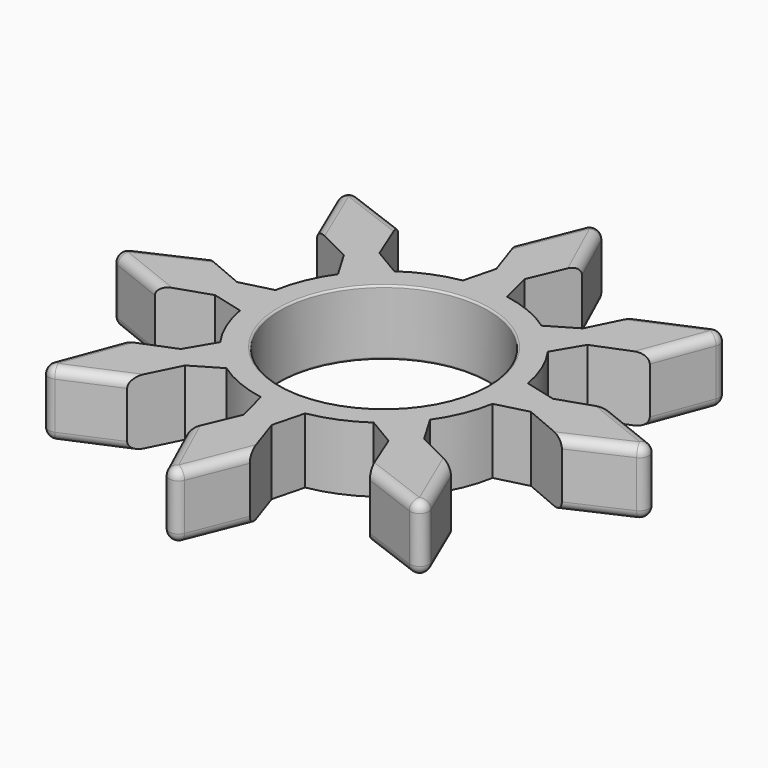
from build123d import *

# Parameters (mm, degrees)
F0_R         = 11.15
F1_DEPTH     = 7
F2_T1_DEPTH  = 13.6241967353
F2_T3_DEPTH  = 13.6241967353
F2_T5_DEPTH  = 13.6241967353
F2_T7_DEPTH  = 13.6241967353
F2_T9_DEPTH  = 13.6241967353
F2_T11_DEPTH = 13.6241967353
F2_T13_DEPTH = 13.6241967353
F3_T1_DEPTH  = 8.9632694004
F3_T3_DEPTH  = 8.9632694004
F3_T5_DEPTH  = 8.9632694004
F3_T7_DEPTH  = 8.9632694004
F3_T9_DEPTH  = 8.9632694004
F3_T11_DEPTH = 8.9632694004
F3_T13_DEPTH = 13.8051316922
F3_T15_DEPTH = 8.9632694004
F3_T17_DEPTH = 11.8546557295
F3_T22_DEPTH = 1
F3_T28_DEPTH = 1
F3_T34_DEPTH = 1
F3_T40_DEPTH = 1
F3_T46_DEPTH = 1
F3_T52_DEPTH = 1
F3_T58_DEPTH = 1
F4_R         = 1
F5_T1_DEPTH  = 8.7823344436
F5_T3_DEPTH  = 5
F5_T8_DEPTH  = 1
F5_T14_DEPTH = 1
F6_R         = 0.2


# Not quite as in the source:
# - a fillet or chamfer that OpenCascade refuses, or shapes differently, is made with other operations: its cross-section is extruded or revolved along the edge and cut away or added


with BuildPart() as f1:
    # F0 (on Top) → F1 (new body)
    with BuildSketch(Plane.XY):
        with BuildLine():
            ThreePointArc((2.3756959996, 13.5358058293), (0.0020367359, 13.7427059484), (-2.3716837507, 13.5365094141))
            ThreePointArc((-2.3716837507, 13.5365094141), (-5.2572241837, 12.6973841721), (-7.8913893394, 11.2511308421))
            ThreePointArc((-7.8913893394, 11.2511308421), (-9.7161203782, 9.7190007577), (-11.2487912633, 7.8947239373))
            ThreePointArc((-11.2487912633, 7.8947239373), (-12.695825322, 5.2609875809), (-13.5358058293, 2.3756959996))
            ThreePointArc((-13.5358058293, 2.3756959996), (-13.7427059484, 0.0020367359), (-13.5365094141, -2.3716837507))
            ThreePointArc((-13.5365094141, -2.3716837507), (-12.6973841721, -5.2572241837), (-11.2511308421, -7.8913893394))
            ThreePointArc((-11.2511308421, -7.8913893394), (-9.7190007577, -9.7161203782), (-7.8947239373, -11.2487912633))
            ThreePointArc((-7.8947239373, -11.2487912633), (-5.2609875809, -12.695825322), (-2.3756959996, -13.5358058293))
            ThreePointArc((-2.3756959996, -13.5358058293), (-0.0020367359, -13.7427059484), (2.3716837507, -13.5365094141))
            ThreePointArc((2.3716837507, -13.5365094141), (5.2572241837, -12.6973841721), (7.8913893394, -11.2511308421))
            ThreePointArc((7.8913893394, -11.2511308421), (9.7161203782, -9.7190007577), (11.2487912633, -7.8947239373))
            ThreePointArc((11.2487912633, -7.8947239373), (12.695825322, -5.2609875809), (13.5358058293, -2.3756959996))
            ThreePointArc((13.5358058293, -2.3756959996), (13.6908833218, -1.192344246), (13.7427060993, 0))
            ThreePointArc((13.7427060993, 0), (13.6910598827, 1.1903151774), (13.5365094141, 2.3716837507))
            ThreePointArc((13.5365094141, 2.3716837507), (12.6973841721, 5.2572241837), (11.2511308421, 7.8913893394))
            ThreePointArc((11.2511308421, 7.8913893394), (9.7190007577, 9.7161203782), (7.8947239373, 11.2487912633))
            ThreePointArc((7.8947239373, 11.2487912633), (5.2609875809, 12.695825322), (2.3756959996, 13.5358058293))
        make_face()
        Circle(F0_R, mode=Mode.SUBTRACT)
        with BuildLine():
            ThreePointArc((-13.5365094141, -2.3716837507), (-13.7427059484, 0.0020367359), (-13.5358058293, 2.3756959996))
            Line((-13.5358058293, 2.3756959996), (-16.9547849556, 1.5))
            Line((-16.9547849556, 1.5), (-21.9830603232, 3.6412940468))
            Line((-21.9830603232, 3.6412940468), (-30, 0))
            Line((-30, 0), (-21.9935868419, -3.2053264533))
            Line((-21.9935868419, -3.2053264533), (-16.923192294, -1.4996672643))
            Line((-16.923192294, -1.4996672643), (-13.5365094141, -2.3716837507))
        make_face()
        with BuildLine():
            ThreePointArc((-11.2487912633, 7.8947239373), (-9.7161203782, 9.7190007577), (-7.8913893394, 11.2511308421))
            Line((-7.8913893394, 11.2511308421), (-10.9281832439, 13.0495035874))
            Line((-10.9281832439, 13.0495035874), (-12.969587313, 18.1191547385))
            Line((-12.969587313, 18.1191547385), (-21.2132034356, 21.2132034356))
            Line((-21.2132034356, 21.2132034356), (-17.8183224696, 13.2853063275))
            Line((-17.8183224696, 13.2853063275), (-13.0269289226, 10.9060791383))
            Line((-13.0269289226, 10.9060791383), (-11.2487912633, 7.8947239373))
        make_face()
        with BuildLine():
            Line((3.6412940468, 21.9830603232), (0, 30))
            Line((0, 30), (-3.2053264533, 21.9935868419))
            Line((-3.2053264533, 21.9935868419), (-1.4996672643, 16.923192294))
            Line((-1.4996672643, 16.923192294), (-2.3716837507, 13.5365094141))
            ThreePointArc((-2.3716837507, 13.5365094141), (0.0020367359, 13.7427059484), (2.3756959996, 13.5358058293))
            Line((2.3756959996, 13.5358058293), (1.5, 16.9547849556))
            Line((1.5, 16.9547849556), (3.6412940468, 21.9830603232))
        make_face()
        with BuildLine():
            Line((10.9060791383, 13.0269289226), (7.8947239373, 11.2487912633))
            ThreePointArc((7.8947239373, 11.2487912633), (9.7190007577, 9.7161203782), (11.2511308421, 7.8913893394))
            Line((11.2511308421, 7.8913893394), (13.0495035874, 10.9281832439))
            Line((13.0495035874, 10.9281832439), (18.1191547385, 12.969587313))
            Line((18.1191547385, 12.969587313), (21.2132034356, 21.2132034356))
            Line((21.2132034356, 21.2132034356), (13.2853063275, 17.8183224696))
            Line((13.2853063275, 17.8183224696), (10.9060791383, 13.0269289226))
        make_face()
        with BuildLine():
            Line((16.923192294, 1.4996672643), (13.5365094141, 2.3716837507))
            ThreePointArc((13.5365094141, 2.3716837507), (13.6910598827, 1.1903151774), (13.7427060993, 0))
            ThreePointArc((13.7427060993, 0), (13.6908833218, -1.192344246), (13.5358058293, -2.3756959996))
            Line((13.5358058293, -2.3756959996), (16.9547849556, -1.5))
            Line((16.9547849556, -1.5), (21.9830603232, -3.6412940468))
            Line((21.9830603232, -3.6412940468), (30, 0))
            Line((30, 0), (21.9935868419, 3.2053264533))
            Line((21.9935868419, 3.2053264533), (16.923192294, 1.4996672643))
        make_face()
        with BuildLine():
            Line((13.0269289226, -10.9060791383), (11.2487912633, -7.8947239373))
            ThreePointArc((11.2487912633, -7.8947239373), (9.7161203782, -9.7190007577), (7.8913893394, -11.2511308421))
            Line((7.8913893394, -11.2511308421), (10.9281832439, -13.0495035874))
            Line((10.9281832439, -13.0495035874), (12.969587313, -18.1191547385))
            Line((12.969587313, -18.1191547385), (21.2132034356, -21.2132034356))
            Line((21.2132034356, -21.2132034356), (17.8183224696, -13.2853063275))
            Line((17.8183224696, -13.2853063275), (13.0269289226, -10.9060791383))
        make_face()
        with BuildLine():
            ThreePointArc((2.3716837507, -13.5365094141), (-0.0020367359, -13.7427059484), (-2.3756959996, -13.5358058293))
            Line((-2.3756959996, -13.5358058293), (-1.5, -16.9547849556))
            Line((-1.5, -16.9547849556), (-3.6412940468, -21.9830603232))
            Line((-3.6412940468, -21.9830603232), (0, -30))
            Line((0, -30), (3.2053264533, -21.9935868419))
            Line((3.2053264533, -21.9935868419), (1.4996672643, -16.923192294))
            Line((1.4996672643, -16.923192294), (2.3716837507, -13.5365094141))
        make_face()
        with BuildLine():
            ThreePointArc((-7.8947239373, -11.2487912633), (-9.7190007577, -9.7161203782), (-11.2511308421, -7.8913893394))
            Line((-11.2511308421, -7.8913893394), (-13.0495035874, -10.9281832439))
            Line((-13.0495035874, -10.9281832439), (-18.1191547385, -12.969587313))
            Line((-18.1191547385, -12.969587313), (-21.2132034356, -21.2132034356))
            Line((-21.2132034356, -21.2132034356), (-13.2853063275, -17.8183224696))
            Line((-13.2853063275, -17.8183224696), (-10.9060791383, -13.0269289226))
            Line((-10.9060791383, -13.0269289226), (-7.8947239373, -11.2487912633))
        make_face()
    extrude(amount=F1_DEPTH)

    # F2: fillet of radius 1 on 7 edges, made by hand

    # F2_s2 → F2_t1 (cut)
    with BuildSketch(Plane(origin=(-28.1768322846, 11.2804503226, 0), x_dir=(0, 0, 1), z_dir=(0.9283662472, -0.3716666667, 0))):
        with BuildLine():
            ThreePointArc((6, 11.15), (6.7071067812, 10.8571067812), (7, 10.15))
            Line((7, 10.15), (7, 11.15))
            Line((7, 11.15), (6, 11.15))
        make_face()
    extrude(amount=F2_T1_DEPTH, mode=Mode.SUBTRACT)

    # F2_s4 → F2_t3 (cut)
    with BuildSketch(Plane(origin=(-11.9475462628, 27.9005120988, 0), x_dir=(0, 0, 1), z_dir=(0.3936460485, -0.9192620891, 0))):
        with BuildLine():
            ThreePointArc((6, 11.15), (6.7071067812, 10.8571067812), (7, 10.15))
            Line((7, 10.15), (7, 11.15))
            Line((7, 11.15), (6, 11.15))
        make_face()
    extrude(amount=F2_T3_DEPTH, mode=Mode.SUBTRACT)

    # F2_s6 → F2_t5 (cut)
    with BuildSketch(Plane(origin=(11.2804503226, 28.1768322846, 0), x_dir=(0, 0, 1), z_dir=(-0.3716666667, -0.9283662472, 0))):
        with BuildLine():
            ThreePointArc((6, 11.15), (6.7071067812, 10.8571067812), (7, 10.15))
            Line((7, 10.15), (7, 11.15))
            Line((7, 11.15), (6, 11.15))
        make_face()
    extrude(amount=F2_T5_DEPTH, mode=Mode.SUBTRACT)

    # F2_s8 → F2_t7 (cut)
    with BuildSketch(Plane(origin=(27.9005120988, 11.9475462628, 0), x_dir=(0, 0, 1), z_dir=(-0.9192620891, -0.3936460485, 0))):
        with BuildLine():
            ThreePointArc((6, 11.15), (6.7071067812, 10.8571067812), (7, 10.15))
            Line((7, 10.15), (7, 11.15))
            Line((7, 11.15), (6, 11.15))
        make_face()
    extrude(amount=F2_T7_DEPTH, mode=Mode.SUBTRACT)

    # F2_s10 → F2_t9 (cut)
    with BuildSketch(Plane(origin=(28.1768322846, -11.2804503226, 0), x_dir=(0, 0, 1), z_dir=(-0.9283662472, 0.3716666667, 0))):
        with BuildLine():
            ThreePointArc((6, 11.15), (6.7071067812, 10.8571067812), (7, 10.15))
            Line((7, 10.15), (7, 11.15))
            Line((7, 11.15), (6, 11.15))
        make_face()
    extrude(amount=F2_T9_DEPTH, mode=Mode.SUBTRACT)

    # F2_s12 → F2_t11 (cut)
    with BuildSketch(Plane(origin=(11.9475462628, -27.9005120988, 0), x_dir=(0, 0, 1), z_dir=(-0.3936460485, 0.9192620891, 0))):
        with BuildLine():
            ThreePointArc((6, 11.15), (6.7071067812, 10.8571067812), (7, 10.15))
            Line((7, 10.15), (7, 11.15))
            Line((7, 11.15), (6, 11.15))
        make_face()
    extrude(amount=F2_T11_DEPTH, mode=Mode.SUBTRACT)

    # F2_s14 → F2_t13 (cut)
    with BuildSketch(Plane(origin=(-11.2804503226, -28.1768322846, 0), x_dir=(0, 0, 1), z_dir=(0.3716666667, 0.9283662472, 0))):
        with BuildLine():
            ThreePointArc((6, 11.15), (6.7071067812, 10.8571067812), (7, 10.15))
            Line((7, 10.15), (7, 11.15))
            Line((7, 11.15), (6, 11.15))
        make_face()
    extrude(amount=F2_T13_DEPTH, mode=Mode.SUBTRACT)

    # F3: fillet of radius 1 on 8 edges, made by hand

    # F3_s2 → F3_t1 (cut)
    with BuildSketch(Plane(origin=(-14.9884732198, 5.6255732129, 0), x_dir=(0, 0, 1), z_dir=(-0.9362286006, 0.35139153, 0))):
        with BuildLine():
            ThreePointArc((7, 11.4062677563), (6.7071067812, 12.1133745375), (6, 12.4062677563))
            Line((6, 12.4062677563), (7, 12.4062677563))
            Line((7, 12.4062677563), (7, 11.4062677563))
        make_face()
    extrude(amount=F3_T1_DEPTH, mode=Mode.SUBTRACT)

    # F3_s4 → F3_t3 (cut)
    with BuildSketch(Plane(origin=(-6.6205700864, 14.5763320202, 0), x_dir=(0, 0, 1), z_dir=(-0.4135422585, 0.910484926, 0))):
        with BuildLine():
            ThreePointArc((7, 11.4062677563), (6.7071067812, 12.1133745375), (6, 12.4062677563))
            Line((6, 12.4062677563), (7, 12.4062677563))
            Line((7, 12.4062677563), (7, 11.4062677563))
        make_face()
    extrude(amount=F3_T3_DEPTH, mode=Mode.SUBTRACT)

    # F3_s6 → F3_t5 (cut)
    with BuildSketch(Plane(origin=(5.6255732129, 14.9884732198, 0), x_dir=(0, 0, 1), z_dir=(0.35139153, 0.9362286006, 0))):
        with BuildLine():
            ThreePointArc((7, 11.4062677563), (6.7071067812, 12.1133745375), (6, 12.4062677563))
            Line((6, 12.4062677563), (7, 12.4062677563))
            Line((7, 12.4062677563), (7, 11.4062677563))
        make_face()
    extrude(amount=F3_T5_DEPTH, mode=Mode.SUBTRACT)

    # F3_s8 → F3_t7 (cut)
    with BuildSketch(Plane(origin=(14.5763320202, 6.6205700864, 0), x_dir=(0, 0, 1), z_dir=(0.910484926, 0.4135422585, 0))):
        with BuildLine():
            ThreePointArc((7, 11.4062677563), (6.7071067812, 12.1133745375), (6, 12.4062677563))
            Line((6, 12.4062677563), (7, 12.4062677563))
            Line((7, 12.4062677563), (7, 11.4062677563))
        make_face()
    extrude(amount=F3_T7_DEPTH, mode=Mode.SUBTRACT)

    # F3_s10 → F3_t9 (cut)
    with BuildSketch(Plane(origin=(14.9884732198, -5.6255732129, 0), x_dir=(0, 0, 1), z_dir=(0.9362286006, -0.35139153, 0))):
        with BuildLine():
            ThreePointArc((7, 11.4062677563), (6.7071067812, 12.1133745375), (6, 12.4062677563))
            Line((6, 12.4062677563), (7, 12.4062677563))
            Line((7, 12.4062677563), (7, 11.4062677563))
        make_face()
    extrude(amount=F3_T9_DEPTH, mode=Mode.SUBTRACT)

    # F3_s12 → F3_t11 (cut)
    with BuildSketch(Plane(origin=(6.6205700864, -14.5763320202, 0), x_dir=(0, 0, 1), z_dir=(0.4135422585, -0.910484926, 0))):
        with BuildLine():
            ThreePointArc((7, 11.4062677563), (6.7071067812, 12.1133745375), (6, 12.4062677563))
            Line((6, 12.4062677563), (7, 12.4062677563))
            Line((7, 12.4062677563), (7, 11.4062677563))
        make_face()
    extrude(amount=F3_T11_DEPTH, mode=Mode.SUBTRACT)

    # F3_s14 → F3_t13 (cut)
    with BuildSketch(Plane(origin=(-5.6255732129, -14.9884732198, 0), x_dir=(0, 0, 1), z_dir=(-0.35139153, -0.9362286006, 0))):
        with BuildLine():
            ThreePointArc((7, 11.4062677563), (6.7071067812, 12.1133745375), (6, 12.4062677563))
            Line((6, 12.4062677563), (7, 12.4062677563))
            Line((7, 12.4062677563), (7, 11.4062677563))
        make_face()
    extrude(amount=F3_T13_DEPTH, mode=Mode.SUBTRACT)

    # F3_s16 → F3_t15 (cut)
    with BuildSketch(Plane(origin=(-14.5763320202, -6.6205700864, 0), x_dir=(0, 0, 1), z_dir=(-0.910484926, -0.4135422585, 0))):
        with BuildLine():
            ThreePointArc((7, 11.4062677563), (6.7071067812, 12.1133745375), (6, 12.4062677563))
            Line((6, 12.4062677563), (7, 12.4062677563))
            Line((7, 12.4062677563), (7, 11.4062677563))
        make_face()
    extrude(amount=F3_T15_DEPTH, mode=Mode.SUBTRACT)

    # F3_s18 → F3_t17 (cut)
    with BuildSketch(Plane.XY.offset(-5.8546557295)):
        with BuildLine():
            ThreePointArc((-27.8677696847, 0.9684590213), (-28.4539682292, 0.0352073057), (-27.8258940928, -0.8703921518))
            Line((-27.8258940928, -0.8703921518), (-30, 0))
            Line((-30, 0), (-27.8677696847, 0.9684590213))
        make_face()
        with BuildLine():
            ThreePointArc((-0.9684590213, -27.8677696847), (-0.0352073057, -28.4539682292), (0.8703921518, -27.8258940928))
            Line((0.8703921518, -27.8258940928), (0, -30))
            Line((0, -30), (-0.9684590213, -27.8677696847))
        make_face()
        with BuildLine():
            ThreePointArc((19.0206849793, -20.3902928619), (20.0950985619, -20.1448892111), (20.2913385984, -19.0604182128))
            Line((20.2913385984, -19.0604182128), (21.2132034356, -21.2132034356))
            Line((21.2132034356, -21.2132034356), (19.0206849793, -20.3902928619))
        make_face()
        with BuildLine():
            ThreePointArc((27.8677696847, -0.9684590213), (28.4539682292, -0.0352073057), (27.8258940928, 0.8703921518))
            Line((27.8258940928, 0.8703921518), (30, 0))
            Line((30, 0), (27.8677696847, -0.9684590213))
        make_face()
        with BuildLine():
            ThreePointArc((20.3902928619, 19.0206849793), (20.1448892111, 20.0950985619), (19.0604182128, 20.2913385984))
            Line((19.0604182128, 20.2913385984), (21.2132034356, 21.2132034356))
            Line((21.2132034356, 21.2132034356), (20.3902928619, 19.0206849793))
        make_face()
        with BuildLine():
            ThreePointArc((0.9684590213, 27.8677696847), (0.0352073057, 28.4539682292), (-0.8703921518, 27.8258940928))
            Line((-0.8703921518, 27.8258940928), (0, 30))
            Line((0, 30), (0.9684590213, 27.8677696847))
        make_face()
        with BuildLine():
            ThreePointArc((-19.0206849793, 20.3902928619), (-20.0950985619, 20.1448892111), (-20.2913385984, 19.0604182128))
            Line((-20.2913385984, 19.0604182128), (-21.2132034356, 21.2132034356))
            Line((-21.2132034356, 21.2132034356), (-19.0206849793, 20.3902928619))
        make_face()
    extrude(amount=F3_T17_DEPTH, mode=Mode.SUBTRACT)


with BuildPart() as f3_tool20:
    # F3_s21 → F3_t22 (new body)
    with BuildSketch(Plane.XY.offset(6)):
        Polygon((-27.4542274261, 0.0579740954), (-27.8677696847, 0.9684590213), (-30, 0), (-27.8258940928, -0.8703921518), align=None)
    extrude(amount=F3_T22_DEPTH)

    # F3_s23 → F3_t24 (revolve, cut)
    with BuildSketch(Plane(origin=(-27.4542274261, 0.0579740954, 6), x_dir=(0.9997408031, 0.0227667896, 0), z_dir=(0.0227667896, -0.9997408031, 0))):
        with BuildLine():
            ThreePointArc((0, -1), (1, 0), (0, 1))
            Line((0, 1), (0, -1))
        make_face()
    revolve(axis=Axis((-27.4542274261, 0.0579740954, 6), (0, 0, 1)), mode=Mode.SUBTRACT)


with BuildPart() as f1_1:
    add(f1.part)

    # F3_t19: cut F3_tool20
    add(f3_tool20.part, mode=Mode.SUBTRACT)


with BuildPart() as f3_tool26:
    # F3_s27 → F3_t28 (new body)
    with BuildSketch(Plane.XY.offset(6)):
        Polygon((-0.0579740954, -27.4542274261), (-0.9684590213, -27.8677696847), (0, -30), (0.8703921518, -27.8258940928), align=None)
    extrude(amount=F3_T28_DEPTH)

    # F3_s29 → F3_t30 (revolve, cut)
    with BuildSketch(Plane(origin=(-0.0579740954, -27.4542274261, 6), x_dir=(-0.0227667896, 0.9997408031, 0), z_dir=(0.9997408031, 0.0227667896, 0))):
        with BuildLine():
            ThreePointArc((0, -1), (1, 0), (0, 1))
            Line((0, 1), (0, -1))
        make_face()
    revolve(axis=Axis((-0.0579740954, -27.4542274261, 6), (0, 0, 1)), mode=Mode.SUBTRACT)


with BuildPart() as f1_2:
    add(f1_1.part)

    # F3_t25: cut F3_tool26
    add(f3_tool26.part, mode=Mode.SUBTRACT)


with BuildPart() as f3_tool32:
    # F3_s33 → F3_t34 (new body)
    with BuildSketch(Plane.XY.offset(6)):
        Polygon((19.3720765093, -19.4540642612), (20.2913385984, -19.0604182128), (21.2132034356, -21.2132034356), (19.0206849793, -20.3902928619), align=None)
    extrude(amount=F3_T34_DEPTH)

    # F3_s35 → F3_t36 (revolve, cut)
    with BuildSketch(Plane(origin=(19.3720765093, -19.4540642612, 6), x_dir=(-0.7230220526, 0.6908249499, 0), z_dir=(0.6908249499, 0.7230220526, 0))):
        with BuildLine():
            ThreePointArc((0, -1), (1, 0), (0, 1))
            Line((0, 1), (0, -1))
        make_face()
    revolve(axis=Axis((19.3720765093, -19.4540642612, 6), (0, 0, 1)), mode=Mode.SUBTRACT)


with BuildPart() as f1_3:
    add(f1_2.part)

    # F3_t31: cut F3_tool32
    add(f3_tool32.part, mode=Mode.SUBTRACT)


with BuildPart() as f3_tool38:
    # F3_s39 → F3_t40 (new body)
    with BuildSketch(Plane.XY.offset(6)):
        Polygon((27.4542274261, -0.0579740954), (27.8677696847, -0.9684590213), (30, 0), (27.8258940928, 0.8703921518), align=None)
    extrude(amount=F3_T40_DEPTH)

    # F3_s41 → F3_t42 (revolve, cut)
    with BuildSketch(Plane(origin=(27.4542274261, -0.0579740954, 6), x_dir=(-0.9997408031, -0.0227667896, 0), z_dir=(-0.0227667896, 0.9997408031, 0))):
        with BuildLine():
            ThreePointArc((0, -1), (1, 0), (0, 1))
            Line((0, 1), (0, -1))
        make_face()
    revolve(axis=Axis((27.4542274261, -0.0579740954, 6), (0, 0, 1)), mode=Mode.SUBTRACT)


with BuildPart() as f1_4:
    add(f1_3.part)

    # F3_t37: cut F3_tool38
    add(f3_tool38.part, mode=Mode.SUBTRACT)


with BuildPart() as f3_tool44:
    # F3_s45 → F3_t46 (new body)
    with BuildSketch(Plane.XY.offset(6)):
        Polygon((19.4540642612, 19.3720765093), (20.3902928619, 19.0206849793), (21.2132034356, 21.2132034356), (19.0604182128, 20.2913385984), align=None)
    extrude(amount=F3_T46_DEPTH)

    # F3_s47 → F3_t48 (revolve, cut)
    with BuildSketch(Plane(origin=(19.4540642612, 19.3720765093, 6), x_dir=(-0.6908249499, -0.7230220526, 0), z_dir=(-0.7230220526, 0.6908249499, 0))):
        with BuildLine():
            ThreePointArc((0, -1), (1, 0), (0, 1))
            Line((0, 1), (0, -1))
        make_face()
    revolve(axis=Axis((19.4540642612, 19.3720765093, 6), (0, 0, 1)), mode=Mode.SUBTRACT)


with BuildPart() as f1_5:
    add(f1_4.part)

    # F3_t43: cut F3_tool44
    add(f3_tool44.part, mode=Mode.SUBTRACT)


with BuildPart() as f3_tool50:
    # F3_s51 → F3_t52 (new body)
    with BuildSketch(Plane.XY.offset(6)):
        Polygon((0.0579740954, 27.4542274261), (0.9684590213, 27.8677696847), (0, 30), (-0.8703921518, 27.8258940928), align=None)
    extrude(amount=F3_T52_DEPTH)

    # F3_s53 → F3_t54 (revolve, cut)
    with BuildSketch(Plane(origin=(0.0579740954, 27.4542274261, 6), x_dir=(0.0227667896, -0.9997408031, 0), z_dir=(-0.9997408031, -0.0227667896, 0))):
        with BuildLine():
            ThreePointArc((0, -1), (1, 0), (0, 1))
            Line((0, 1), (0, -1))
        make_face()
    revolve(axis=Axis((0.0579740954, 27.4542274261, 6), (0, 0, 1)), mode=Mode.SUBTRACT)


with BuildPart() as f1_6:
    add(f1_5.part)

    # F3_t49: cut F3_tool50
    add(f3_tool50.part, mode=Mode.SUBTRACT)


with BuildPart() as f3_tool56:
    # F3_s57 → F3_t58 (new body)
    with BuildSketch(Plane.XY.offset(6)):
        Polygon((-19.3720765093, 19.4540642612), (-19.0206849793, 20.3902928619), (-21.2132034356, 21.2132034356), (-20.2913385984, 19.0604182128), align=None)
    extrude(amount=F3_T58_DEPTH)

    # F3_s59 → F3_t60 (revolve, cut)
    with BuildSketch(Plane(origin=(-19.3720765093, 19.4540642612, 6), x_dir=(0.7230220526, -0.6908249499, 0), z_dir=(-0.6908249499, -0.7230220526, 0))):
        with BuildLine():
            ThreePointArc((0, -1), (1, 0), (0, 1))
            Line((0, 1), (0, -1))
        make_face()
    revolve(axis=Axis((-19.3720765093, 19.4540642612, 6), (0, 0, 1)), mode=Mode.SUBTRACT)


with BuildPart() as f1_7:
    add(f1_6.part)

    # F3_t55: cut F3_tool56
    add(f3_tool56.part, mode=Mode.SUBTRACT)

    # F4
    f4_edges = [f1_7.edges().sort_by_distance(p)[0] for p in [
        (19.254724, 15.995136, 0),
        (2.304877, 24.925415, 0),
        (-15.995136, 19.254724, 0),
        (-24.925415, 2.304877, 0),
        (-19.666179, -17.091395, 0),
        (-2.304877, -24.925415, 0),
        (15.995136, -19.254724, 0),
        (24.925415, -2.304877, 0),
    ]]
    fillet(f4_edges, radius=F4_R)

    # F5: fillet of radius 1 on 3 edges, made by hand

    # F5_s2 → F5_t1 (cut)
    with BuildSketch(Plane(origin=(-23.4495716531, -10.0415663045, 0), x_dir=(0, 0, 1), z_dir=(0.9192620891, 0.3936460485, 0))):
        with BuildLine():
            ThreePointArc((7, 10.15), (6.7071067812, 10.8571067812), (6, 11.15))
            Line((6, 11.15), (7, 11.15))
            Line((7, 11.15), (7, 10.15))
        make_face()
        with BuildLine():
            ThreePointArc((0, 10.15), (0.2928932188, 10.8571067812), (1, 11.15))
            Line((1, 11.15), (0, 11.15))
            Line((0, 11.15), (0, 10.15))
        make_face()
    extrude(amount=F5_T1_DEPTH, mode=Mode.SUBTRACT)

    # F5_s4 → F5_t3 (cut)
    with BuildSketch(Plane.XY.offset(1)):
        with BuildLine():
            ThreePointArc((-19.0604182128, -20.2913385984), (-20.1448892111, -20.0950985619), (-20.3902928619, -19.0206849793))
            Line((-20.3902928619, -19.0206849793), (-21.2132034356, -21.2132034356))
            Line((-21.2132034356, -21.2132034356), (-19.0604182128, -20.2913385984))
        make_face()
    extrude(amount=F5_T3_DEPTH, mode=Mode.SUBTRACT)


with BuildPart() as f5_tool6:
    # F5_s7 → F5_t8 (new body)
    with BuildSketch(Plane.XY.offset(1)):
        Polygon((-19.4540642612, -19.3720765093), (-20.3902928619, -19.0206849793), (-21.2132034356, -21.2132034356), (-19.0604182128, -20.2913385984), align=None)
    extrude(amount=-F5_T8_DEPTH)

    # F5_s9 → F5_t10 (revolve, cut)
    with BuildSketch(Plane(origin=(-19.4540642612, -19.3720765093, 1), x_dir=(0.6908249499, 0.7230220526, 0), z_dir=(-0.7230220526, 0.6908249499, 0))):
        with BuildLine():
            ThreePointArc((0, -1), (1, 0), (0, 1))
            Line((0, 1), (0, -1))
        make_face()
    revolve(axis=Axis((-19.4540642612, -19.3720765093, 1), (0, 0, -1)), mode=Mode.SUBTRACT)


with BuildPart() as f1_8:
    add(f1_7.part)

    # F5_t5: cut F5_tool6
    add(f5_tool6.part, mode=Mode.SUBTRACT)


with BuildPart() as f5_tool12:
    # F5_s13 → F5_t14 (new body)
    with BuildSketch(Plane.XY.offset(6)):
        Polygon((-19.4540642612, -19.3720765093), (-20.3902928619, -19.0206849793), (-21.2132034356, -21.2132034356), (-19.0604182128, -20.2913385984), align=None)
    extrude(amount=F5_T14_DEPTH)

    # F5_s15 → F5_t16 (revolve, cut)
    with BuildSketch(Plane(origin=(-19.4540642612, -19.3720765093, 6), x_dir=(0.6908249499, 0.7230220526, 0), z_dir=(0.7230220526, -0.6908249499, 0))):
        with BuildLine():
            ThreePointArc((0, -1), (1, 0), (0, 1))
            Line((0, 1), (0, -1))
        make_face()
    revolve(axis=Axis((-19.4540642612, -19.3720765093, 6), (0, 0, 1)), mode=Mode.SUBTRACT)


with BuildPart() as f1_9:
    add(f1_8.part)

    # F5_t11: cut F5_tool12
    add(f5_tool12.part, mode=Mode.SUBTRACT)

    # F6
    f6_edges = [f1_9.edges().sort_by_distance(p)[0] for p in [
        (-11.15, 0, 7),
        (-11.15, 0, 0),
    ]]
    fillet(f6_edges, radius=F6_R)


solid = f1_9.part
